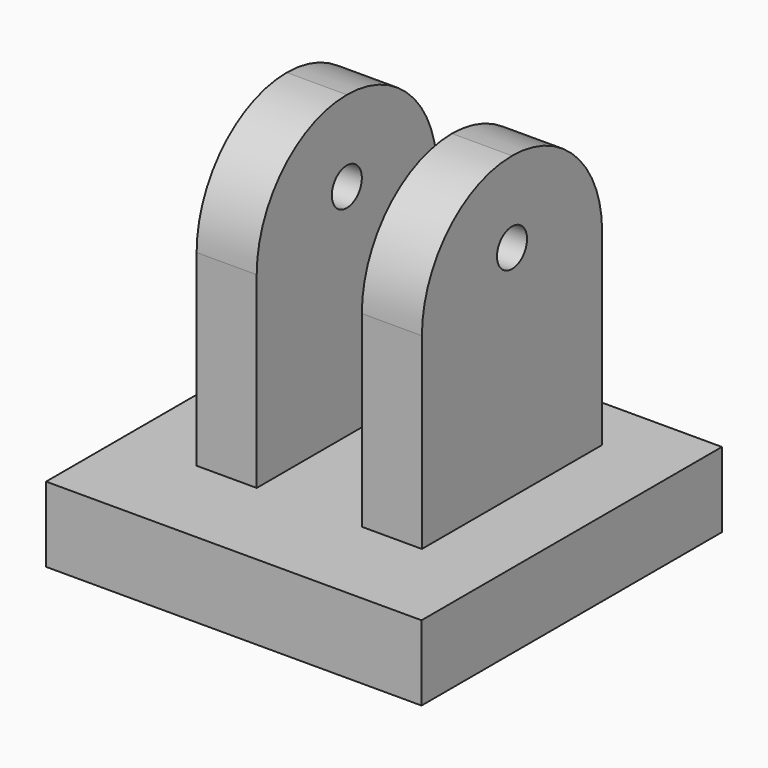
from build123d import *

# Parameters (mm, degrees)
F0_W     = 50
F0_H     = 50
F1_DEPTH = 10
F2_W     = 8
F2_H     = 30
F3_DEPTH = 40
F4_R     = 14.99999
F6_D     = 5


# Not quite as in the source:
# - a fillet or chamfer is up to 0.001 mm smaller than in the source, because OpenCascade refuses the exact size


with BuildPart() as f1:
    # F0 (on Top) → F1 (new body)
    with BuildSketch(Plane.XY):
        with Locations((2.6419349015, 1.5731524348)):
            Rectangle(F0_W, F0_H)
    extrude(amount=F1_DEPTH)

    # F2 (on face) → F3 (join)
    with BuildSketch(Plane.XY.offset(10)):
        with Locations((-8.3580650985, 4.1337611525)):
            Rectangle(F2_W, F2_H)
        with Locations((13.6419349015, 4.1337611525)):
            Rectangle(F2_W, F2_H)
    extrude(amount=F3_DEPTH)

    # F4 (radius 15 in the source; OpenCascade refuses exactly that, so slightly less here)
    f4_edges = [f1.edges().sort_by_distance(p)[0] for p in [
        (13.641935, -10.866239, 50),
        (13.641935, 19.133761, 50),
        (-8.358065, 19.133761, 50),
        (-8.358065, -10.866239, 50),
    ]]
    fillet(f4_edges, radius=F4_R)

    # F6 (through all)
    with Locations(Plane(origin=(-12.3580650985, 0, 0), x_dir=(0, -1, 0), z_dir=(-1, 0, 0))):
        with Locations((-4.1337611525, 39.2225831747)):
            Hole(F6_D / 2)


solid = f1.part
